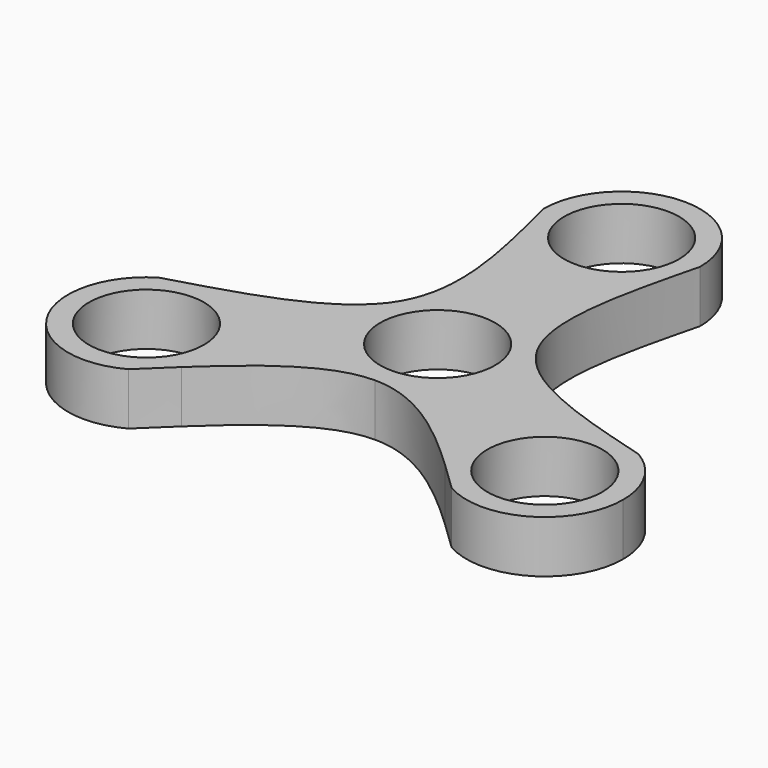
from build123d import *

# Parameters (mm, degrees)
F0_R     = 11
F1_DEPTH = 10


# Not quite as in the source:
# - ends of sketch curves that miss each other by under 0.0002 mm in the source are joined


with BuildPart() as f1:
    # F0 (on Top) → F1 (new body)
    with BuildSketch(Plane.XY):
        with BuildLine():
            add(Edge.make_bspline(
                [(-45.9731322266, -9.229160229), (-43.4071259384, -8.4900716571), (-40.8523723257, -7.7580834253), (-38.3590158595, -7.002148962)],
                knots=[0, 0, 0, 0, 0.0911278571, 0.0911278571, 0.0911278571, 0.0911278571], degree=3))
            ThreePointArc((-45.9731322266, -9.229160229), (-51.0954988233, -29.5), (-30.9792533273, -35.1993202853))
            add(Edge.make_bspline(
                [(-30.9792533273, -35.1993202853), (-29.0552189861, -33.3450108014), (-27.1429808317, -31.496831403), (-25.2406198636, -29.713928552)],
                knots=[0, 0, 0, 0, 0.0911399969, 0.0911399969, 0.0911399969, 0.0911399969], degree=3))
            ThreePointArc((-25.2406198636, -29.713928552), (-23.6488480446, -26.0020326995), (-23.1051177665, -22))
            ThreePointArc((-23.1051177665, -22), (-27.5886656888, -11.3040084285), (-38.3590158595, -7.002148962))
        make_face()
        with Locations((-38.1051177665, -22)):
            Circle(F0_R, mode=Mode.SUBTRACT)
        with BuildLine():
            add(Edge.make_bspline(
                [(-38.3590158595, -7.002148962), (-27.1330019101, -3.5986521316), (-17.1515902552, 0.2902668448), (-12.9914200153, 7.4981996163)],
                knots=[0.0911278571, 0.0911278571, 0.0911278571, 0.0911278571, 0.5014192088, 0.5014192088, 0.5014192088, 0.5014192088], degree=3))
            ThreePointArc((-38.3590158595, -7.002148962), (-27.5886656888, -11.3040084285), (-23.1051177665, -22))
            ThreePointArc((-23.1051177665, -22), (-23.6488480446, -26.0020326995), (-25.2406198636, -29.713928552))
            add(Edge.make_bspline(
                [(-25.2406198636, -29.713928552), (-16.6860428704, -21.6965333438), (-8.3311964125, -14.9991213274), (-0.001581884, -14.9999997526)],
                knots=[0.0911399969, 0.0911399969, 0.0911399969, 0.0911399969, 0.5009802604, 0.5009802604, 0.5009802604, 0.5009802604], degree=3))
            ThreePointArc((-0.001581884, -14.9999997526), (-12.9902568617, -7.5002151081), (-12.9914200153, 7.4981996163))
        make_face()
        with BuildLine():
            add(Edge.make_bspline(
                [(-12.9914200153, 7.4981996163), (-12.9910736554, 7.4987997212), (-8.7775182768, 14.8003583601), (-10.5373469555, 25.5076949363), (-13.2795920522, 37.0248702573)],
                knots=[0.5014192088, 0.5014192088, 0.5014192088, 0.5014192088, 0.5014533681, 0.9170240175, 0.9170240175, 0.9170240175, 0.9170240175], degree=3))
            ThreePointArc((-12.9914200153, 7.4981996163), (-0.000790756, 14.9999999792), (12.9906296223, 7.4995694554))
            add(Edge.make_bspline(
                [(13.2855190223, 37.0361659764), (10.5442311657, 25.5033031012), (8.7843940058, 14.7858120219), (12.9905467554, 7.4997129635), (12.9906296223, 7.4995694554)],
                knots=[0.082935592, 0.082935592, 0.082935592, 0.082935592, 0.499552834, 0.4995610405, 0.4995610405, 0.4995610405, 0.4995610405], degree=3))
            ThreePointArc((13.2855190223, 37.0361659764), (0.0063781315, 29.000001356), (-13.2795920522, 37.0248702573))
        make_face()
        with BuildLine():
            ThreePointArc((12.9906296223, 7.4995694554), (-0.000790756, 14.9999999792), (-12.9914202607, 7.498199758))
            ThreePointArc((-12.9914202607, 7.498199758), (-12.9902568617, -7.5002151081), (-0.001581884, -14.9999999166))
            ThreePointArc((-0.001581884, -14.9999999166), (10.6060424226, -10.6071609835), (15, 0))
            ThreePointArc((15, 0), (14.4889517277, 3.8820455732), (12.9906296223, 7.4995694554))
        make_face()
        Circle(F0_R, mode=Mode.SUBTRACT)
        with BuildLine():
            ThreePointArc((15, 0), (10.6060424226, -10.6071609835), (-0.001581884, -14.9999999166))
            add(Edge.make_bspline(
                [(-0.001581884, -14.9999999166), (-0.0010545892, -14.9999998083), (8.4030291654, -15.0013139041), (16.7814390471, -21.8215724341), (25.3649320041, -29.9175543408)],
                knots=[0.5009802604, 0.5009802604, 0.5009802604, 0.5009802604, 0.5010062047, 0.9144846967, 0.9144846967, 0.9144846967, 0.9144846967], degree=3))
            ThreePointArc((25.3649320041, -29.9175543408), (25.119350955, -14.4920135645), (38.6102651526, -7.008508209))
            add(Edge.make_bspline(
                [(12.9906296082, 7.4995694472), (17.1802492182, 0.2423799612), (27.2886260541, -3.6105886019), (38.6102651526, -7.008508209)],
                knots=[0.4995610405, 0.4995610405, 0.4995610405, 0.4995610405, 0.914537264, 0.914537264, 0.914537264, 0.914537264], degree=3))
            ThreePointArc((12.9906296082, 7.4995694472), (14.4889517277, 3.8820455732), (15, 0))
        make_face()
        with BuildLine():
            add(Edge.make_bspline(
                [(-13.2795920522, 37.0248702573), (-13.8271294721, 39.3244766884), (-14.4138387907, 41.6564041587), (-15, 44)],
                knots=[0.9170240175, 0.9170240175, 0.9170240175, 0.9170240175, 1, 1, 1, 1], degree=3))
            ThreePointArc((-13.2795920522, 37.0248702573), (0.0063781315, 29.000001356), (13.2855190223, 37.0361659764))
            add(Edge.make_bspline(
                [(15, 44), (14.4158248487, 41.6601580392), (13.8312245488, 39.3320018523), (13.2855190223, 37.0361659764)],
                knots=[0, 0, 0, 0, 0.082935592, 0.082935592, 0.082935592, 0.082935592], degree=3))
            ThreePointArc((15, 44), (0, 59), (-15, 44))
        make_face()
        with Locations((0, 44)):
            Circle(F0_R, mode=Mode.SUBTRACT)
        with BuildLine():
            ThreePointArc((38.6102651526, -7.008508209), (25.119350955, -14.4920135645), (25.3649320041, -29.9175543408))
            add(Edge.make_bspline(
                [(25.3649320041, -29.9175543408), (27.1401634065, -31.5919590833), (28.9241895579, -33.3209501687), (30.7190564774, -35.055500704)],
                knots=[0.9144846967, 0.9144846967, 0.9144846967, 0.9144846967, 1, 1, 1, 1], degree=3))
            ThreePointArc((30.7190564774, -35.055500704), (45.6618723829, -34.9574480384), (53.1051177665, -22))
            ThreePointArc((53.1051177665, -22), (51.1281832536, -14.5568981387), (45.7184823908, -9.0757329377))
            add(Edge.make_bspline(
                [(38.6102651526, -7.008508209), (40.9419126032, -7.7082965101), (43.3250191135, -8.3887844569), (45.7184823908, -9.0757329377)],
                knots=[0.914537264, 0.914537264, 0.914537264, 0.914537264, 1, 1, 1, 1], degree=3))
        make_face()
        with Locations((38.1051177665, -22)):
            Circle(F0_R, mode=Mode.SUBTRACT)
    extrude(amount=F1_DEPTH)


solid = f1.part
